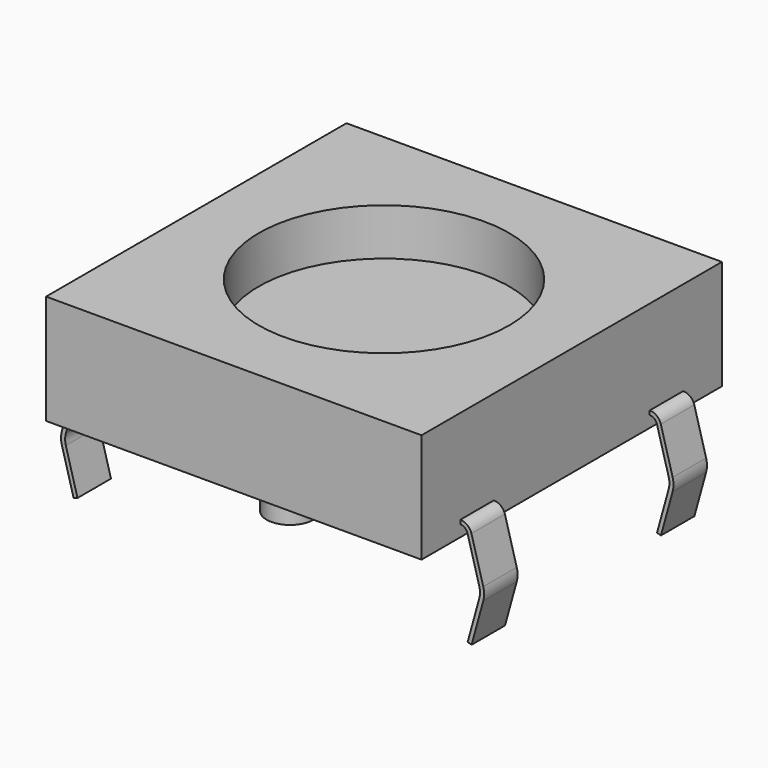
from build123d import *

# Parameters (mm, degrees)
F0_W     = 12
F0_H     = 12
F1_DEPTH = 3.5
F2_R     = 4
F3_DEPTH = 1.5
F4_R     = 0.75
F5_DEPTH = 1.5
F6_W     = 1.3371782843
F6_H     = 0.1306298655


with BuildPart() as f1:
    # F0 (on Top) → F1 (new body)
    with BuildSketch(Plane.XY):
        Rectangle(F0_W, F0_H)
    extrude(amount=-F1_DEPTH)

    # F2 (on Top) → F3 (cut)
    with BuildSketch(Plane.XY):
        Circle(F2_R)
    extrude(amount=-F3_DEPTH, mode=Mode.SUBTRACT)

    # F4 (on face) → F5 (join)
    with BuildSketch(Plane(origin=(0, 0, -3.5), x_dir=(1, 0, 0), z_dir=(0, 0, -1))):
        with Locations((0, -3.75)):
            Circle(F4_R)
        with Locations((0, 3.75)):
            Circle(F4_R)
    extrude(amount=F5_DEPTH)

    # F8: sweep along a path in F7
    with BuildLine(Plane(origin=(0, 6, 0), x_dir=(-1, 0, 0), z_dir=(0, 1, 0))) as f8_path:
        ThreePointArc((-6, -2.9808722661), (-6.2386599526, -3.0614322815), (-6.3796732575, -3.2701515593))
        Line((-6.3796732575, -3.2701515593), (-6.7573431879, -4.6420912258))
        ThreePointArc((-6.7573431879, -4.6420912258), (-6.7854382425, -4.8500061966), (-6.7573431879, -5.0579211675))
        Line((-6.7573431879, -5.0579211675), (-6.3840173786, -6.4140801969))
    # F6 (on face) → F8 (sweep)
    with BuildSketch(Plane.YZ.offset(6)):
        with Locations((-3.7832342787, -3.070783685)):
            Rectangle(F6_W, F6_H)
        with Locations((3.7832342787, -3.070783685)):
            Rectangle(F6_W, F6_H)
    sweep(path=f8_path.line)

    # F9: F1 across plane


with BuildPart() as f1_1:
    add(f1.part)
    add(f1.part.mirror(Plane.YZ))


solid = f1_1.part
